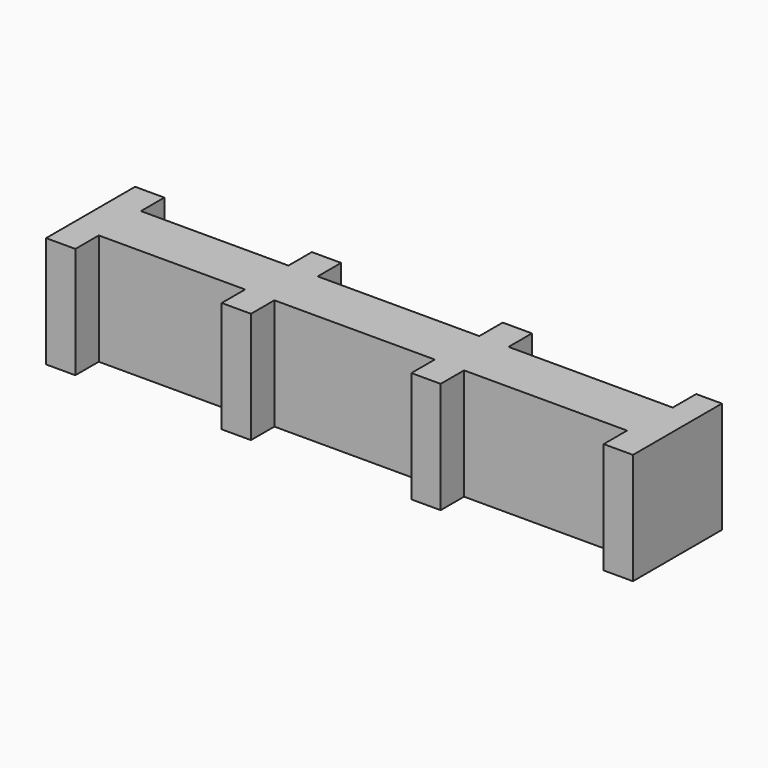
from build123d import *

# Parameters (mm, degrees)
F0_W           = 200.5
F0_H           = 38
F1_DEPTH       = 38
F2_W           = 55.7
F2_H           = 38
F2_W_2         = 54.8
F2_W_3         = 50
F3_DEPTH       = 10
F4_W           = 50.4
F4_H           = 38
F4_W_2         = 55.2
F4_W_3         = 56.1
F4_H_2         = 38.1344797201
F5_DEPTH       = 10
F6_TEXT_SIZE   = 5.5828416306
F6_TEXT_SIZE_2 = 9.2238252465
F7_DEPTH       = 1.5


# Not quite as in the source:
# - Text() gives the source's letters only with a copy of the font that has no kerning and outlines rounded to 1/6400 em; it was checked with that copy


with BuildPart() as f1:
    # F0 (on Front) → F1 (new body)
    with BuildSketch(Plane.XZ):
        with Locations((100.25, -19)):
            Rectangle(F0_W, F0_H)
    extrude(amount=F1_DEPTH)

    # F2 (on face) → F3 (cut)
    with BuildSketch(Plane.XZ.offset(38)):
        with Locations((162.65, -19)):
            Rectangle(F2_W, F2_H)
        with Locations((97.4, -19)):
            Rectangle(F2_W_2, F2_H)
        with Locations((35, -19)):
            Rectangle(F2_W_3, F2_H)
    extrude(amount=-F3_DEPTH, mode=Mode.SUBTRACT)

    # F4 (on face) → F5 (cut)
    with BuildSketch(Plane(origin=(0, 0, 0), x_dir=(-1, 0, 0), z_dir=(0, 1, 0))):
        with Locations((-35.2, -19)):
            Rectangle(F4_W, F4_H)
        with Locations((-98, -19)):
            Rectangle(F4_W_2, F4_H)
        with Locations((-163.65, -18.9327601399)):
            Rectangle(F4_W_3, F4_H_2)
    extrude(amount=-F5_DEPTH, mode=Mode.SUBTRACT)

    # F6 (on face) → F7 (cut)
    with BuildSketch(Plane(origin=(0, 0, -38), x_dir=(1, 0, 0), z_dir=(0, 0, -1))):
        with Locations((69.8407515883, 21.0684742779)):
            Text('No Go', F6_TEXT_SIZE, font='Open Sans', text_align=(TextAlign.LEFT, TextAlign.BOTTOM))
        with Locations((79.2781785131, 11.6310426965)):
            Text('Go', F6_TEXT_SIZE_2, font='Open Sans', text_align=(TextAlign.LEFT, TextAlign.BOTTOM))
    extrude(amount=-F7_DEPTH, mode=Mode.SUBTRACT)


solid = f1.part
